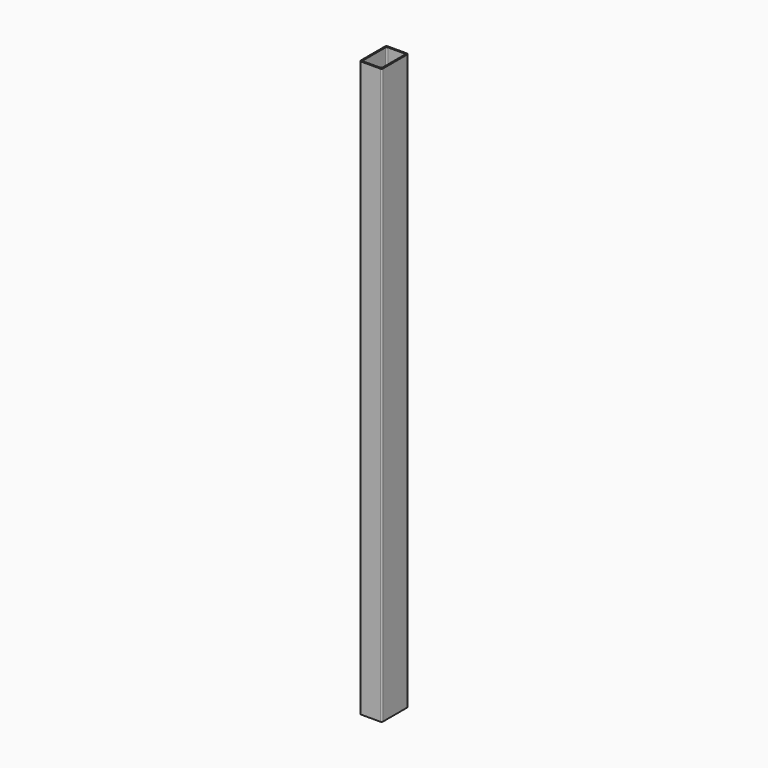
from build123d import *

# Parameters (mm, degrees)
F0_W     = 50.8
F0_H     = 76.2
F0_W_2   = 44.45
F0_H_2   = 69.85
F2_DEPTH = 1320.8
F3_R     = 3.175


# Not quite as in the source:
# - a variable given as a bare number and used for a length is read in inches; the dataset says mm whatever the document's units were


with BuildPart() as f2:
    # F0 (on Top) → F2 (new body)
    with BuildSketch(Plane.XY):
        Rectangle(F0_W, F0_H)
        Rectangle(F0_W_2, F0_H_2, mode=Mode.SUBTRACT)
    extrude(amount=F2_DEPTH)

    # F3
    f3_edges = [f2.edges().sort_by_distance(p)[0] for p in [
        (25.4, 38.1, 660.4),
        (-25.4, 38.1, 660.4),
        (25.4, -38.1, 660.4),
        (22.225, -34.925, 660.4),
        (-22.225, -34.925, 660.4),
        (-22.225, 34.925, 660.4),
        (22.225, 34.925, 660.4),
        (-25.4, -38.1, 660.4),
    ]]
    fillet(f3_edges, radius=F3_R)


solid = f2.part
